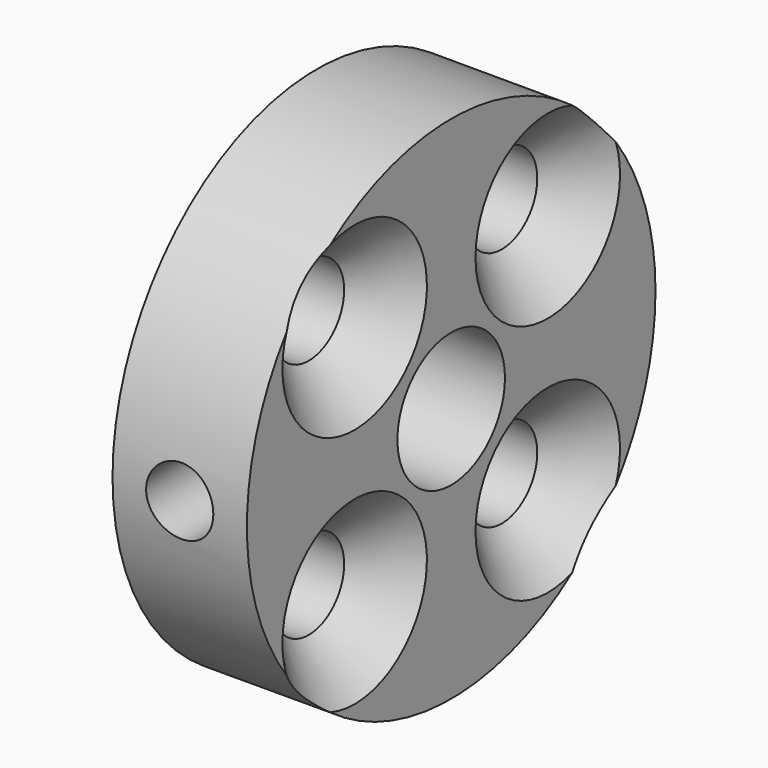
from build123d import *

# Parameters (mm, degrees)
F0_R           = 9.5
F0_R_2         = 2.5
F1_DEPTH       = 2.5
F3_R           = 1.25
F4_DEPTH       = 9.501
F5_D           = 3.3
F5_CSINK_D     = 6.72
F5_CSINK_ANGLE = 90


with BuildPart() as f1:
    # F0 (on Right) → F1 (new body, symmetric)
    with BuildSketch(Plane.YZ):
        Circle(F0_R)
        Circle(F0_R_2, mode=Mode.SUBTRACT)
    extrude(amount=F1_DEPTH, both=True)

    # F3 (on Front) → F4 (cut, through all)
    with BuildSketch(Plane.XZ):
        Circle(F3_R)
    extrude(amount=F4_DEPTH, mode=Mode.SUBTRACT)

    # F5 (through all)
    with Locations(Plane.YZ.offset(2.5)):
        with Locations((-4.4901280605, 4.4901280605), (4.4901280605, 4.4901280605), (4.4901280605, -4.4901280605), (-4.4901280605, -4.4901280605)):
            CounterSinkHole(F5_D / 2, F5_CSINK_D / 2, counter_sink_angle=F5_CSINK_ANGLE)


solid = f1.part
